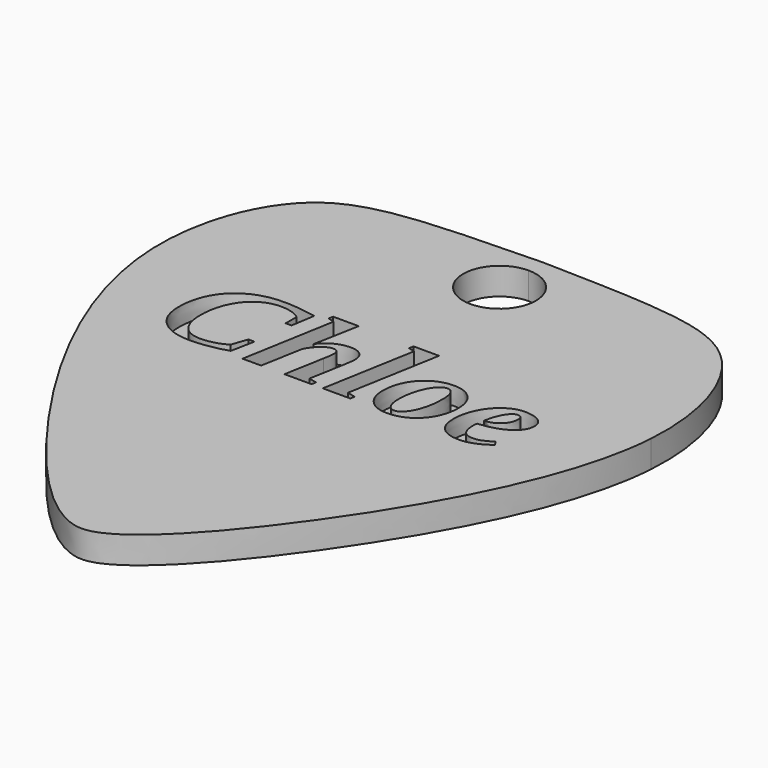
from build123d import *

# Parameters (mm, degrees)
F1_DEPTH     = 1.5
F2_TEXT_SIZE = 7.9746073526
F3_DEPTH     = 1


# Not quite as in the source:
# - Text() gives the source's letters only with a copy of the font that has no kerning and outlines rounded to 1/6400 em; it was checked with that copy


with BuildPart() as f1:
    # F0 (on Top) → F1 (new body)
    with BuildSketch(Plane.XY):
        with BuildLine():
            add(Edge.make_bspline(
                [(0, 0), (-1.9324692099, 0), (-9.0020229041, 8.0092222642), (-15.5290450329, 21.2111688172), (-12.1408436083, 31.6617431719), (-6.9365538313, 31.8392763808), (0, 32)],
                knots=[0, 0, 0, 0, 0.2439819692, 0.5356196802, 0.7455018812, 1, 1, 1, 1], degree=3))
            Line((0, 0), (0, 22))
            Line((0, 22), (0, 26.9813453157))
            ThreePointArc((0, 26.9813453157), (-2.0186546843, 29), (0, 31.0186546843))
            Line((0, 31.0186546843), (0, 32))
        make_face()
        with BuildLine():
            Line((0, 22), (0, 0))
            add(Edge.make_bspline(
                [(0, 0), (1.9324692099, 0), (9.0020229041, 8.0092222642), (13.6914832441, 17.4944060967), (14, 22)],
                knots=[0, 0, 0, 0, 0.2439819692, 0.5356196802, 0.5356196802, 0.5356196802, 0.5356196802], degree=3))
            Line((14, 22), (0, 22))
        make_face()
        with BuildLine():
            Line((0, 26.9813453157), (0, 22))
            Line((0, 22), (14, 22))
            add(Edge.make_bspline(
                [(14, 22), (14.2220295022, 25.2425297886), (12.1408436083, 31.6617431719), (6.9365538313, 31.8392763808), (0, 32)],
                knots=[0.5356196802, 0.5356196802, 0.5356196802, 0.5356196802, 0.7455018812, 1, 1, 1, 1], degree=3))
            Line((0, 32), (0, 31.0186546843))
            ThreePointArc((0, 31.0186546843), (1.4274044162, 30.4274044162), (2.0186546843, 29))
            ThreePointArc((2.0186546843, 29), (1.4274044162, 27.5725955838), (0, 26.9813453157))
        make_face()
    extrude(amount=F1_DEPTH)

    # F2 (on face) + F0 (on Top) → F3 (cut)
    with BuildSketch(Plane.XY.offset(1.5)):
        with Locations((-9.9879703484, 16.8056059629)):
            Text('Chloe', F2_TEXT_SIZE, font='Tinos', font_style=FontStyle.BOLDITALIC, text_align=(TextAlign.LEFT, TextAlign.BOTTOM))
    with BuildSketch(Plane.XY):
        with BuildLine():
            add(Edge.make_bspline(
                [(0, 0), (-1.9324692099, 0), (-9.0020229041, 8.0092222642), (-15.5290450329, 21.2111688172), (-12.1408436083, 31.6617431719), (-6.9365538313, 31.8392763808), (0, 32)],
                knots=[0, 0, 0, 0, 0.2439819692, 0.5356196802, 0.7455018812, 1, 1, 1, 1], degree=3))
            Line((0, 0), (0, 22))
            Line((0, 22), (0, 26.9813453157))
            ThreePointArc((0, 26.9813453157), (-2.0186546843, 29), (0, 31.0186546843))
            Line((0, 31.0186546843), (0, 32))
        make_face()
        with BuildLine():
            Line((0, 22), (0, 0))
            add(Edge.make_bspline(
                [(0, 0), (1.9324692099, 0), (9.0020229041, 8.0092222642), (13.6914832441, 17.4944060967), (14, 22)],
                knots=[0, 0, 0, 0, 0.2439819692, 0.5356196802, 0.5356196802, 0.5356196802, 0.5356196802], degree=3))
            Line((14, 22), (0, 22))
        make_face()
        with BuildLine():
            Line((0, 26.9813453157), (0, 22))
            Line((0, 22), (14, 22))
            add(Edge.make_bspline(
                [(14, 22), (14.2220295022, 25.2425297886), (12.1408436083, 31.6617431719), (6.9365538313, 31.8392763808), (0, 32)],
                knots=[0.5356196802, 0.5356196802, 0.5356196802, 0.5356196802, 0.7455018812, 1, 1, 1, 1], degree=3))
            Line((0, 32), (0, 31.0186546843))
            ThreePointArc((0, 31.0186546843), (1.4274044162, 30.4274044162), (2.0186546843, 29))
            ThreePointArc((2.0186546843, 29), (1.4274044162, 27.5725955838), (0, 26.9813453157))
        make_face()
    extrude(amount=-F3_DEPTH, mode=Mode.SUBTRACT)


solid = f1.part
